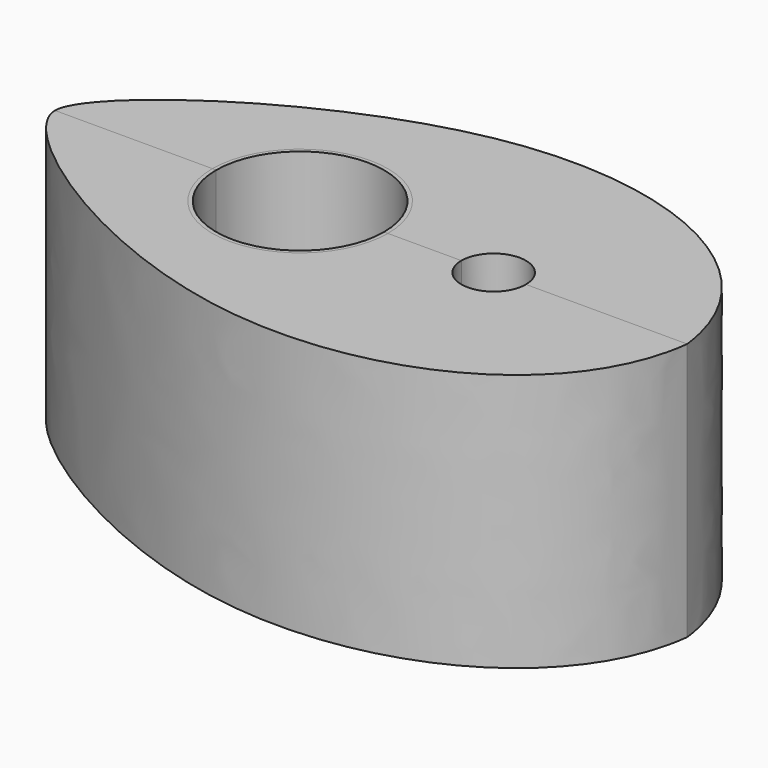
from build123d import *
from build123d import SkipClean  # not in build123d's __all__

# Parameters (mm, degrees)
F1_DEPTH = 20
F3_R     = 6.8
F3_R_2   = 6.5
F4_DEPTH = 20
F5_R     = 4.75
F6_DEPTH = 17


with BuildPart() as f1:
    # F0 (on Top) → F1 (new body)
    with BuildSketch(Plane.XY):
        with BuildLine():
            add(Edge.make_bspline(
                [(-34, 0), (-34.0019650757, 3.3683322836), (-8.8829017766, 21.2695751777), (13.7677686289, 10.092517361), (15, 0)],
                knots=[0, 0, 0, 0, 0.5, 1, 1, 1, 1], degree=3))
            Line((-34, 0), (-21.5, 0))
            ThreePointArc((-21.5, 0), (-15, 6.5), (-8.5, 0))
            Line((-8.5, 0), (-2.5, 0))
            ThreePointArc((-2.5, 0), (0, 2.5), (2.5, 0))
            Line((2.5, 0), (15, 0))
        make_face()
    extrude(amount=F1_DEPTH)

    # F2: F1 across plane


with BuildPart() as f1_1:
    add(f1.part, clean=False)
    with SkipClean():  # cleaning this boolean's faces spoils the solid; the shape is the same uncleaned
        add(f1.part.mirror(Plane.XZ), clean=False)

    # F3 (on Top) → F4 (join)
    with BuildSketch(Plane.XY):
        with Locations((-15, 0)):
            Circle(F3_R)
        with Locations((-15, 0)):
            Circle(F3_R_2, mode=Mode.SUBTRACT)
    with SkipClean():  # cleaning this boolean's faces spoils the solid; the shape is the same uncleaned
        extrude(amount=F4_DEPTH)


with BuildPart() as f6:
    # F5 (on Top) → F6 (new body)
    with BuildSketch(Plane.XY):
        Circle(F5_R)
    extrude(amount=F6_DEPTH)


with BuildPart() as f1_2:
    add(f1_1.part, clean=False)

    # F7: cut F6
    add(f6.part, mode=Mode.SUBTRACT)


solid = f1_2.part
